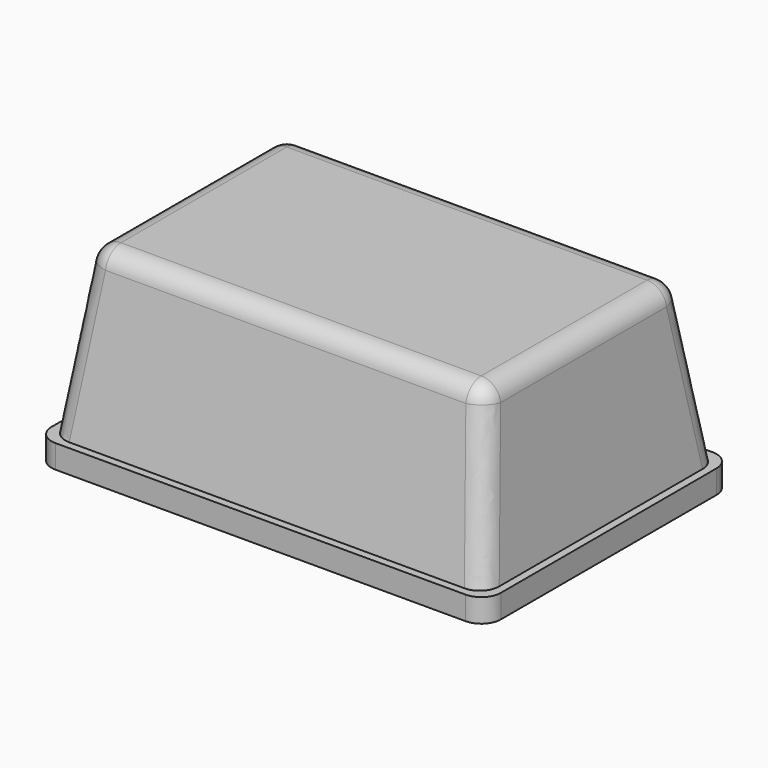
from build123d import *

# Parameters (mm, degrees)
F2_W     = 101.22
F2_H     = 61.63
F0_W     = 111.14
F0_H     = 75.07
F4_R     = 5
F5_T     = 2.5
F7_DEPTH = 6


# Not quite as in the source:
# - a shell that OpenCascade refuses in one call is made with other operations: the cavity is built on its own and cut out


with BuildPart() as f3:
    # F2 (on offset) → F3 section 0
    with BuildSketch(Plane.XY.offset(42)):
        Rectangle(F2_W, F2_H)
    # F0 (on Top) → F3 section 1
    with BuildSketch(Plane.XY):
        Rectangle(F0_W, F0_H)
    loft()

    # F4
    f4_edges = [f3.edges().sort_by_distance(p)[0] for p in [
        (-53.09, 34.175, 21),
        (53.09, 34.175, 21),
        (53.09, -34.175, 21),
        (-53.09, -34.175, 21),
        (0, -30.815, 42),
        (50.61, 0, 42),
        (0, 30.815, 42),
        (-50.61, 0, 42),
    ]]
    fillet(f4_edges, radius=F4_R)

    # F5: shell of thickness 2.5, made by hand


with BuildPart() as f5_core1:
    # F5_t2: copy of F3
    add(f3.part)

    # the walls: a layer under each face that stays
    f5_faces = [f5_core1.faces().sort_by_distance(p)[0] for p in [
        (-53.3506124987, 0, 18.7932006155),
        (-51.8873286605, 33.0489229278, 18.9750242391),
        (-51.8873286605, -33.0489229278, 18.9750242391),
        (-49.4874767675, 0, 40.7371115956),
        (0, 34.5118037996, 18.8949762528),
        (0, -34.5118037996, 18.8949762528),
        (51.8873286605, 33.0489229278, 18.9750242391),
        (51.8873299173, -33.0489246306, 18.9750135967),
        (53.3506124987, 0, 18.7932006155),
        (-48.5145599261, 28.9002335794, 40.7371115784),
        (-48.5145599261, -28.9002335794, 40.7371115784),
        (0, 0, 42),
        (0, 29.7956483786, 40.8045868716),
        (0, -29.7956483786, 40.8045868716),
        (48.5145600153, 28.9002373676, 40.7371091413),
        (48.5145599261, -28.9002335794, 40.7371115784),
        (49.4874767675, 0, 40.7371115956),
    ]]
    thicken(f5_faces, amount=-F5_T, mode=Mode.SUBTRACT)


with BuildPart() as f3_1:
    add(f3.part)

    # what is left inside the walls is the cavity
    f5_cavity = [f5_core1.part.solids().sort_by_distance(p)[0] for p in [
        (10.775811, 15.952675, 0.025),
    ]]
    add(f5_cavity, mode=Mode.SUBTRACT)

    # F6 (on face) → F7 (join)
    with BuildSketch(Plane(origin=(0, 0, 0), x_dir=(1, 0, 0), z_dir=(0, 0, -1))):
        with BuildLine():
            Line((52.57, 39.535), (-52.57, 39.535))
            ThreePointArc((-52.57, 39.535), (-56.1055339059, 38.0705339059), (-57.57, 34.535))
            Line((-57.57, 34.535), (-57.57, -34.535))
            ThreePointArc((-57.57, -34.535), (-56.1055339059, -38.0705339059), (-52.57, -39.535))
            Line((-52.57, -39.535), (52.57, -39.535))
            ThreePointArc((52.57, -39.535), (56.1055339059, -38.0705339059), (57.57, -34.535))
            Line((57.57, -34.535), (57.57, 34.535))
            ThreePointArc((57.57, 34.535), (56.1055339059, 38.0705339059), (52.57, 39.535))
        make_face()
    extrude(amount=F7_DEPTH)


solid = f3_1.part
